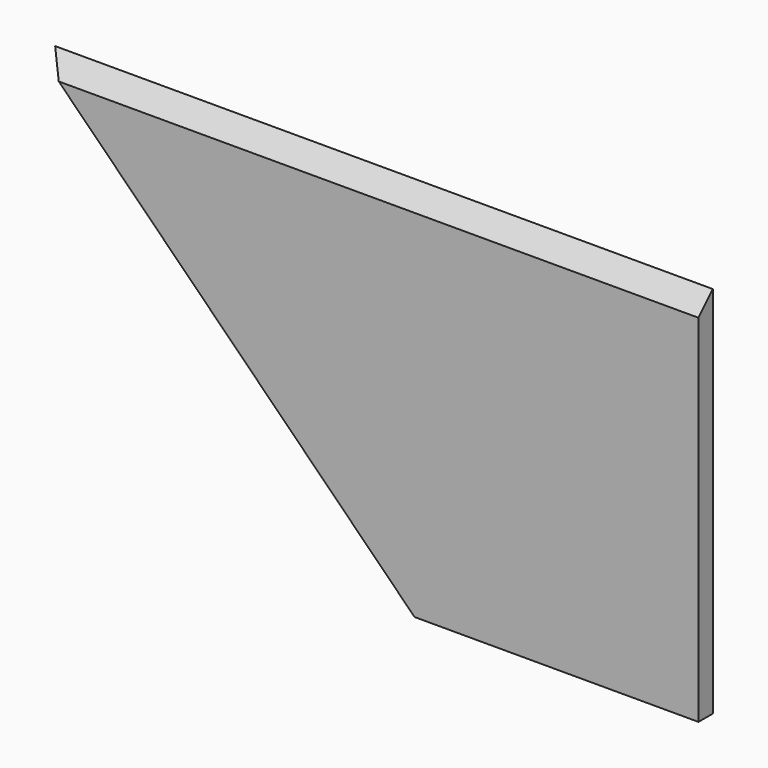
from build123d import *

# Parameters (mm, degrees)
F1_DEPTH = 15.875
F2_SIZE  = 15.87499


# Not quite as in the source:
# - a fillet or chamfer is up to 0.001 mm smaller than in the source, because OpenCascade refuses the exact size


with BuildPart() as f1:
    # F0 (on Front) → F1 (new body)
    with BuildSketch(Plane.XZ):
        Polygon((-250.825, 0), (0, 0), (0, 330.2), (-581.025, 330.2), align=None)
    extrude(amount=F1_DEPTH)

    # F2 (size 15.875 in the source; OpenCascade refuses exactly that, so slightly less here)
    f2_edges = [f1.edges().sort_by_distance(p)[0] for p in [
        (-290.5125, -15.875, 330.2),
    ]]
    chamfer(f2_edges, length=F2_SIZE)


solid = f1.part
